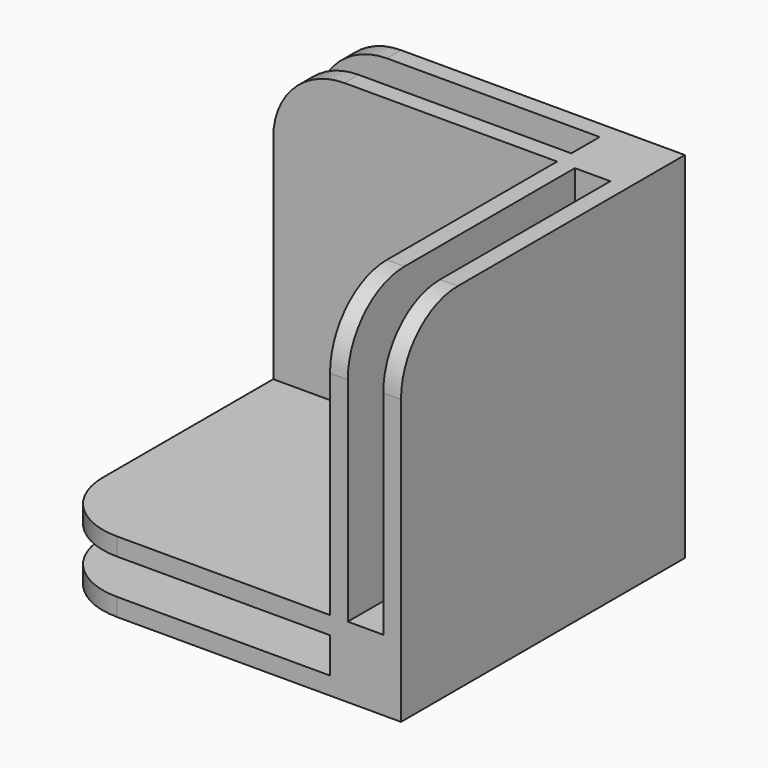
from build123d import *

# Parameters (mm, degrees)
F1_DEPTH = 10
F3_DEPTH = 10
F5_DEPTH = 10
F6_W     = 20
F6_H     = 5
F6_W_2   = 5
F6_H_2   = 30
F6_H_3   = 20
F7_DEPTH = 40
F8_W     = 30
F8_H     = 5
F8_W_2   = 20
F9_DEPTH = 40


# Not quite as in the source:
# - a feature names something its author has since deleted; it is built from what else it names


with BuildPart() as f1:
    # F0 (on Top) → F1 (new body)
    with BuildSketch(Plane.XY):
        with BuildLine():
            Line((0, -50), (0, 0))
            Line((0, 0), (-50, 0))
            Line((-50, 0), (-50, -40))
            ThreePointArc((-50, -40), (-47.0710678119, -47.0710678119), (-40, -50))
            Line((-40, -50), (0, -50))
        make_face()
    extrude(amount=F1_DEPTH)

    # F2 (on Right) → F3 (join)
    with BuildSketch(Plane.YZ):
        with BuildLine():
            Line((-50, 10), (0, 10))
            Line((0, 10), (0, 50))
            Line((0, 50), (-40, 50))
            ThreePointArc((-40, 50), (-47.0710678119, 47.0710678119), (-50, 40))
            Line((-50, 40), (-50, 10))
        make_face()
    extrude(amount=-F3_DEPTH)

    # F4 (on Front) → F5 (join)
    with BuildSketch(Plane.XZ):
        with BuildLine():
            Line((-50, 10), (-10, 10))
            Line((-10, 10), (-10, 50))
            Line((-10, 50), (-40, 50))
            ThreePointArc((-40, 50), (-47.0710678119, 47.0710678119), (-50, 40))
            Line((-50, 40), (-50, 10))
        make_face()
    extrude(amount=F5_DEPTH)

    # F6 (on face) → F7 (cut)
    with BuildSketch(Plane.XZ.offset(50)):
        Polygon((-15, 2.5), (-10, 2.5), (-10, 7.5), (-40, 7.5), (-40, 2.5), align=None)
        with Locations((-50, 5)):
            Rectangle(F6_W, F6_H)
        with Locations((-5, 25)):
            Rectangle(F6_W_2, F6_H_2)
        with Locations((-5, 50)):
            Rectangle(F6_W_2, F6_H_3)
    extrude(amount=-F7_DEPTH, mode=Mode.SUBTRACT)

    # F8 (on face) → F9 (cut)
    with BuildSketch(Plane.XY.offset(50)):
        with Locations((-25, -5)):
            Rectangle(F8_W, F8_H)
        with Locations((-50, -5)):
            Rectangle(F8_W_2, F8_H)
    extrude(amount=-F9_DEPTH, mode=Mode.SUBTRACT)


solid = f1.part
